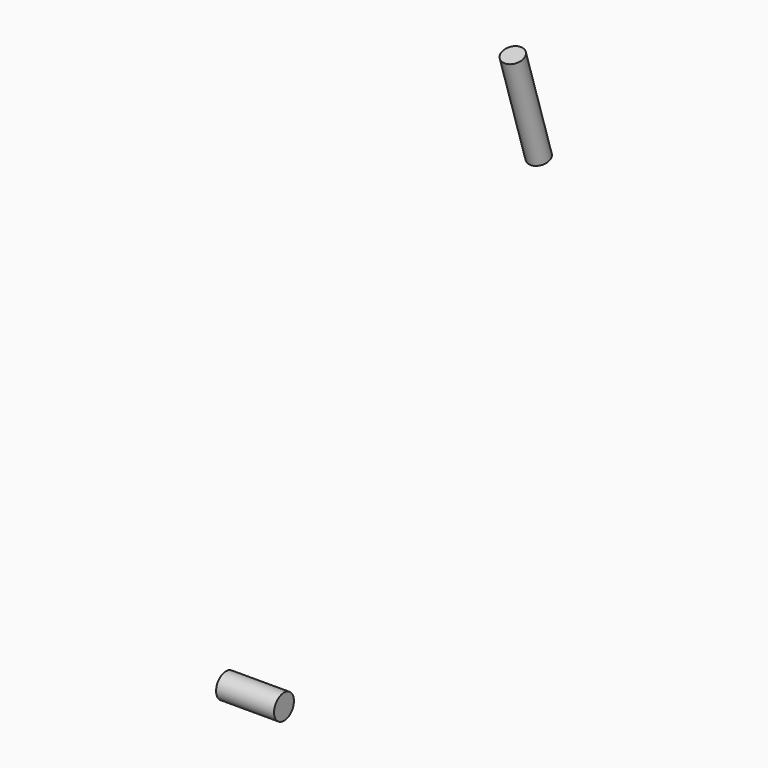
from build123d import *

# Parameters (mm, degrees)
F4_R      = 15
F7_DEPTH  = 35
F9_R      = 12.7
F10_DEPTH = 130


# Not quite as in the source:
# - the program builds the solid bodies; features that only make, move or delete a surface that nothing else refers to are left out


with BuildPart() as f7:
    # F4 (on Right) → F7 (new body, symmetric)
    with BuildSketch(Plane.YZ):
        with Locations((0, 271.5)):
            Circle(F4_R)
    extrude(amount=F7_DEPTH, both=True)


with BuildPart() as f10:
    # F9 (on line) → F10 (new body, through all)
    with BuildSketch(Plane(origin=(0, -192.657256288, 611.0307526806), x_dir=(1, 0, 0), z_dir=(0, 0.3007057995, -0.9537169507))):
        with Locations((0, -609.872031448)):
            Circle(F9_R)
    extrude(amount=F10_DEPTH)


solid = Compound([f7.part, f10.part])
